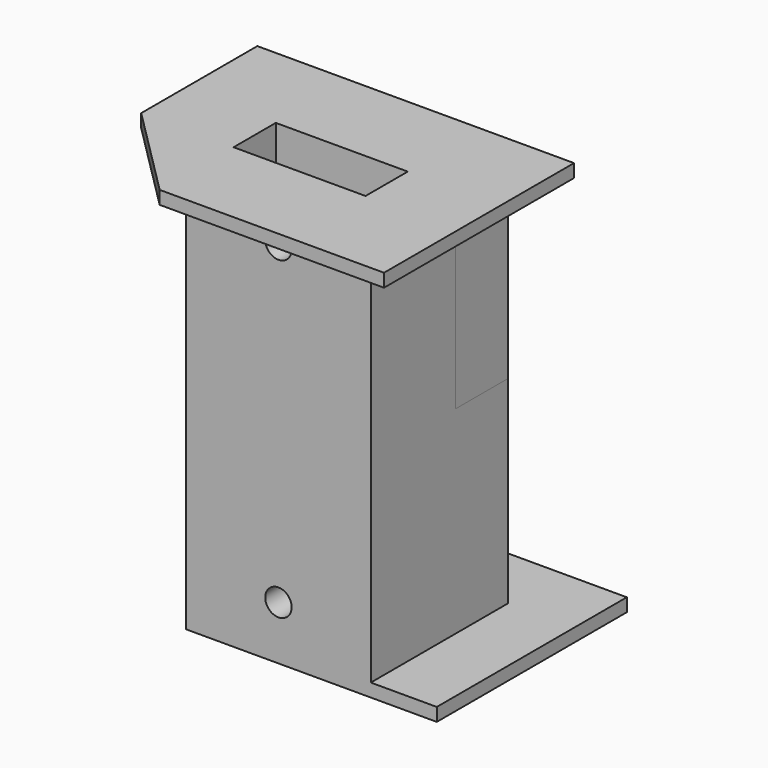
from build123d import *

# Parameters (mm, degrees)
F0_W      = 14
F0_H      = 8
F0_W_2    = 10
F0_H_2    = 4
F1_DEPTH  = 16
F2_W      = 24
F2_H      = 18
F2_W_2    = 14
F2_H_2    = 8
F3_DEPTH  = 1
F4_R      = 1
F5_DEPTH  = 18.001
F6_SIZE   = 7
F9_DEPTH  = 5
F10_DEPTH = 5


with BuildPart() as f1:
    # F0 (on Top) → F1 (new body)
    with BuildSketch(Plane.XY):
        Rectangle(F0_W, F0_H)
        Rectangle(F0_W_2, F0_H_2, mode=Mode.SUBTRACT)
    extrude(amount=-F1_DEPTH)

    # F4 (on face) → F5 (cut, through all)
    with BuildSketch(Plane(origin=(0, 9, 0), x_dir=(-1, 0, 0), z_dir=(0, 1, 0))):
        with BuildLine():
            ThreePointArc((1, -28), (0, -27), (-1, -28))
            Line((-1, -28), (1, -28))
        make_face()
        with BuildLine():
            Line((1, -28), (-1, -28))
            ThreePointArc((-1, -28), (0, -29), (1, -28))
        make_face()
        with Locations((0, -4.0714931674)):
            Circle(F4_R)
    extrude(amount=-F5_DEPTH, mode=Mode.SUBTRACT)


with BuildPart() as f3:
    # F2 (on face) → F3 (new body)
    with BuildSketch(Plane.XY):
        Rectangle(F2_W, F2_H)
        Rectangle(F2_W_2, F2_H_2, mode=Mode.SUBTRACT)
    extrude(amount=-F3_DEPTH)

    # F6
    f6_edges = [f3.edges().sort_by_distance(p)[0] for p in [
        (-12, -9, -0.5),
    ]]
    chamfer(f6_edges, length=F6_SIZE)


with BuildPart() as f7_1:
    # F7: instance of F3
    add(f3.part.mirror(Plane(origin=(0, 0, -16), x_dir=(1, 0, 0), z_dir=(0, 0, -1))))


with BuildPart() as f7_2:
    # F7: instance of F1
    add(f1.part.mirror(Plane(origin=(0, 0, -16), x_dir=(1, 0, 0), z_dir=(0, 0, -1))))


with BuildPart() as f7_2_1:
    # F8: moved
    add(f7_2.part.moved(Location((0, 5, 0))))


with BuildPart() as f7_1_1:
    # F8: moved
    add(f7_1.part.moved(Location((0, 5, 0))))


with BuildPart() as f1_1:
    add(f1.part)

    # F9 (add, through all): a face of the model
    f9_faces = [f7_2_1.part.faces().sort_by_distance(p)[0] for p in [
        (0, 1, -23.9441190926),
    ]]

    add(f7_1_1.part)  # F9 merges F7_1

    add(f7_2_1.part)  # F9 merges F7_2
    extrude(f9_faces, amount=F9_DEPTH)

    # F10 (add, through all): a face of the model
    f10_faces = [f1_1.faces().sort_by_distance(p)[0] for p in [
        (0, 4, -8.0558809074),
    ]]

    add(f3.part)  # F10 merges F3
    extrude(f10_faces, amount=F10_DEPTH)


solid = f1_1.part
